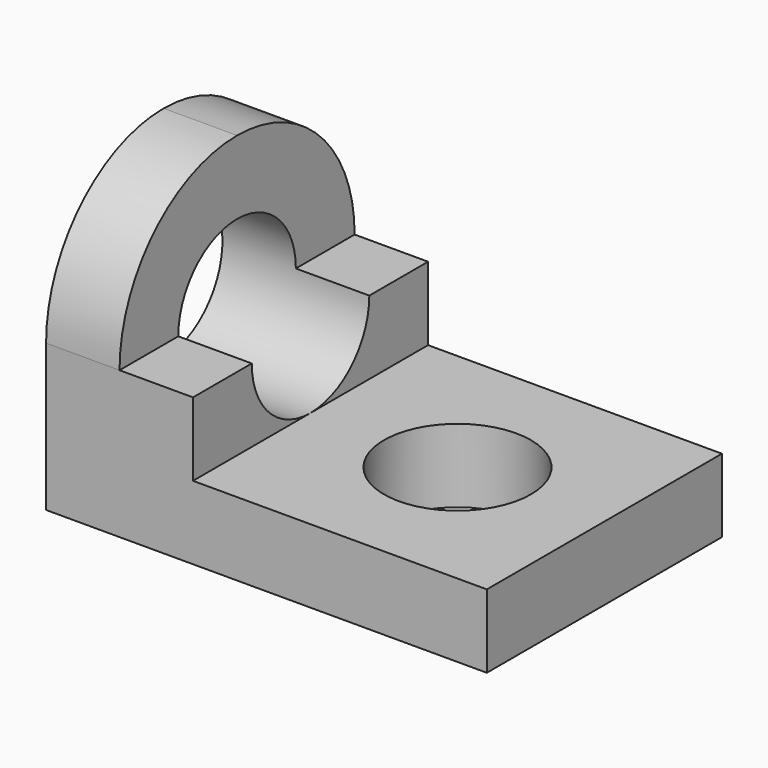
from build123d import *

# Parameters (mm, degrees)
F0_W      = 60
F0_H      = 40
F1_DEPTH  = 10
F2_W      = 10
F2_H      = 40
F3_DEPTH  = 30
F4_W      = 10
F4_H      = 40
F5_DEPTH  = 10
F6_R      = 10
F7_DEPTH  = 60.001
F8_R      = 20
F9_R      = 19.99999
F10_R     = 10
F11_DEPTH = 10.001


# Not quite as in the source:
# - a fillet or chamfer is up to 0.001 mm smaller than in the source, because OpenCascade refuses the exact size


with BuildPart() as f1:
    # F0 (on Top) → F1 (new body)
    with BuildSketch(Plane.XY):
        Rectangle(F0_W, F0_H)
    extrude(amount=F1_DEPTH)

    # F2 (on face) → F3 (join)
    with BuildSketch(Plane.XY.offset(10)):
        with Locations((-25, 0)):
            Rectangle(F2_W, F2_H)
    extrude(amount=F3_DEPTH)

    # F4 (on face) → F5 (join)
    with BuildSketch(Plane.XY.offset(10)):
        with Locations((-15, 0)):
            Rectangle(F4_W, F4_H)
    extrude(amount=F5_DEPTH)

    # F6 (on face) → F7 (cut, through all)
    with BuildSketch(Plane(origin=(-30, 0, 0), x_dir=(0, -1, 0), z_dir=(-1, 0, 0))):
        with Locations((0, 20)):
            Circle(F6_R)
    extrude(amount=-F7_DEPTH, mode=Mode.SUBTRACT)

    # F8
    f8_edges = [f1.edges().sort_by_distance(p)[0] for p in [
        (-25, -20, 40),
    ]]
    fillet(f8_edges, radius=F8_R)

    # F9 (radius 20 in the source; OpenCascade refuses exactly that, so slightly less here)
    f9_edges = [f1.edges().sort_by_distance(p)[0] for p in [
        (-25, 20, 40),
    ]]
    fillet(f9_edges, radius=F9_R)

    # F10 (on face) → F11 (cut, through all)
    with BuildSketch(Plane.XY.offset(10)):
        with Locations((10, 0)):
            Circle(F10_R)
    extrude(amount=-F11_DEPTH, mode=Mode.SUBTRACT)


solid = f1.part
